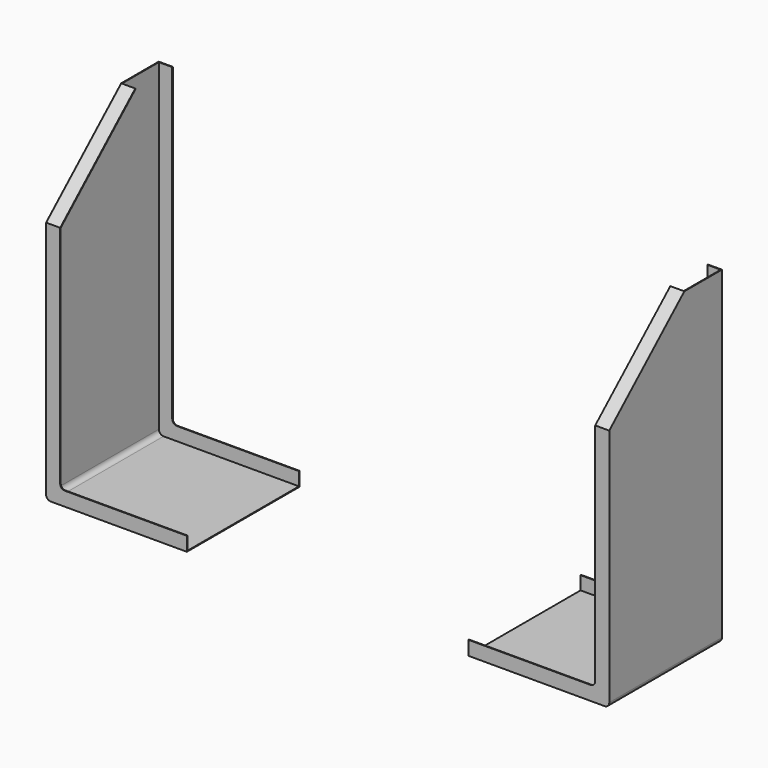
from build123d import *

# Parameters (mm, degrees)
F1_DEPTH = 300
F2_SIZE2 = 180
F2_SIZE  = 200
F4_DEPTH = 1.5
F5_W     = 30
F5_H     = 269.072481
F6_DEPTH = 1.5
F8_DEPTH = 1.5
F9_SIZE2 = 200
F9_SIZE  = 180


with BuildPart() as f1:
    # F0 (on Front) → F1 (new body)
    with BuildSketch(Plane.XZ):
        with BuildLine():
            Line((1.5, 0), (0, 0))
            Line((0, 0), (0, -690))
            ThreePointArc((0, -690), (2.928932, -697.071068), (10, -700))
            Line((10, -700), (300, -700))
            Line((300, -700), (300, -698.5))
            Line((300, -698.5), (11.5, -698.5))
            ThreePointArc((11.5, -698.5), (4.428932, -695.571068), (1.5, -688.5))
            Line((1.5, -688.5), (1.5, 0))
        make_face()
    extrude(amount=F1_DEPTH)

    # F2
    f2_edges = [f1.edges().sort_by_distance(p)[0] for p in [
        (0.75, -300, 0),
    ]]
    f2_side = f1.faces().sort_by_distance((0.75, -150, 0))[0]
    chamfer(f2_edges, length=F2_SIZE, length2=F2_SIZE2, reference=f2_side)

    # F3 (on face) → F4 (join)
    with BuildSketch(Plane.XZ.offset(300)):
        with BuildLine():
            Line((30, -180), (0, -180))
            Line((0, -180), (0, -690))
            ThreePointArc((0, -690), (2.928932, -697.071068), (10, -700))
            Line((10, -700), (300, -700))
            Line((300, -700), (300, -670))
            Line((300, -670), (40, -670))
            ThreePointArc((40, -670), (32.928932, -667.071068), (30, -660))
            Line((30, -660), (30, -180))
        make_face()
    extrude(amount=-F4_DEPTH)

    # F5 (on face) → F6 (join)
    with BuildSketch(Plane(origin=(0, -44.751381, 49.723757), x_dir=(1, 0, 0), z_dir=(0, -0.668965, 0.743294))):
        with Locations((15, -208.865655)):
            Rectangle(F5_W, F5_H)
    extrude(amount=-F6_DEPTH)

    # F7 (on face) → F8 (join)
    with BuildSketch(Plane(origin=(0, 0, 0), x_dir=(-1, 0, 0), z_dir=(0, 1, 0))):
        with BuildLine():
            Line((-300, -670), (-300, -700))
            Line((-300, -700), (-10, -700))
            ThreePointArc((-10, -700), (-2.928932, -697.071068), (0, -690))
            Line((0, -690), (0, 0))
            Line((0, 0), (-30, 0))
            Line((-30, 0), (-30, -660))
            ThreePointArc((-30, -660), (-32.928932, -667.071068), (-40, -670))
            Line((-40, -670), (-300, -670))
        make_face()
    extrude(amount=-F8_DEPTH)


with BuildPart() as f1b:
    # F0 (on Front) → F1, piece 2 (new body)
    with BuildSketch(Plane.XZ):
        with BuildLine():
            Line((900, -700), (1190, -700))
            ThreePointArc((1190, -700), (1197.071068, -697.071068), (1200, -690))
            Line((1200, -690), (1200, 0))
            Line((1200, 0), (1198.5, 0))
            Line((1198.5, 0), (1198.5, -688.5))
            ThreePointArc((1198.5, -688.5), (1195.571068, -695.571068), (1188.5, -698.5))
            Line((1188.5, -698.5), (900, -698.5))
            Line((900, -698.5), (900, -700))
        make_face()
    extrude(amount=F1_DEPTH)

    # F3 (on face) → F4, piece 2 (join)
    with BuildSketch(Plane.XZ.offset(300)):
        with BuildLine():
            Line((900, -670), (900, -700))
            Line((900, -700), (1190, -700))
            ThreePointArc((1190, -700), (1197.071068, -697.071068), (1200, -690))
            Line((1200, -690), (1200, -180))
            Line((1200, -180), (1170, -180))
            Line((1170, -180), (1170, -660))
            ThreePointArc((1170, -660), (1167.071068, -667.071068), (1160, -670))
            Line((1160, -670), (900, -670))
        make_face()
    extrude(amount=-F4_DEPTH)

    # F5 (on face) → F6, piece 2 (join)
    with BuildSketch(Plane(origin=(0, -44.751381, 49.723757), x_dir=(1, 0, 0), z_dir=(0, -0.668965, 0.743294))):
        with Locations((1185, -208.865655)):
            Rectangle(F5_W, F5_H)
    extrude(amount=-F6_DEPTH)

    # F7 (on face) → F8, piece 2 (join)
    with BuildSketch(Plane(origin=(0, 0, 0), x_dir=(-1, 0, 0), z_dir=(0, 1, 0))):
        with BuildLine():
            Line((-1190, -700), (-900, -700))
            Line((-900, -700), (-900, -670))
            Line((-900, -670), (-1160, -670))
            ThreePointArc((-1160, -670), (-1167.071068, -667.071068), (-1170, -660))
            Line((-1170, -660), (-1170, 0))
            Line((-1170, 0), (-1200, 0))
            Line((-1200, 0), (-1200, -690))
            ThreePointArc((-1200, -690), (-1197.071068, -697.071068), (-1190, -700))
        make_face()
    extrude(amount=-F8_DEPTH)

    # F9
    f9_edges = [f1b.edges().sort_by_distance(p)[0] for p in [
        (1199.25, -300, 0),
    ]]
    f9_side = f1b.faces().sort_by_distance((907.615773, -300, -685))[0]
    chamfer(f9_edges, length=F9_SIZE, length2=F9_SIZE2, reference=f9_side)


solid = Compound([f1.part, f1b.part])
